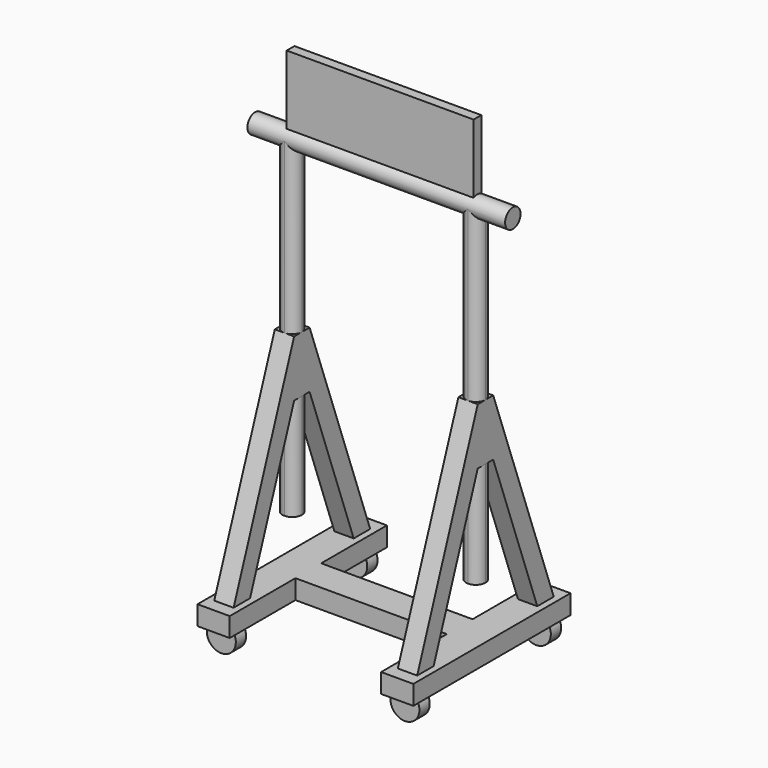
from build123d import *

# Parameters (mm, degrees)
F2_DEPTH          = 3
F6_DEPTH          = 1.5
F9_DEPTH          = 26.2
F9_DEPTH_BACK     = 25
F10_R             = 1.5
F11_DEPTH         = 20
F13_R             = 2.25
F14_DEPTH         = 2
F14_COPIES2_COUNT = 2
F14_COPIES2_PITCH = 38.242646
F15_W             = 29
F15_H             = 11
F16_DEPTH         = 0.75


# Not quite as in the source:
# - a pattern or mirror of a feature is missing from the dataset's text; its kind, count and spacing are read off the source's solid


with BuildPart() as f2:
    # F1 (on offset) → F2 (new body)
    with BuildSketch(Plane.XY.offset(3.5)):
        Polygon((-11.75, -15.25), (-11.75, -2.5), (-11.75, 2.5), (-11.75, 15.25), (-16.75, 15.25), (-16.75, 0), (-16.75, -15.25), align=None)
        Polygon((0, -2.5), (11.75, -2.5), (11.75, 2.5), (0, 2.5), (-11.75, 2.5), (-11.75, -2.5), align=None)
        Polygon((16.75, -15.25), (16.75, 0), (16.75, 15.25), (11.75, 15.25), (11.75, 2.5), (11.75, -2.5), (11.75, -15.25), align=None)
    extrude(amount=F2_DEPTH)

    # F5 (on plane+point) → F6 (join, symmetric)
    with BuildSketch(Plane.YZ.offset(14.25)):
        Polygon((10.057664814, 6.5), (13.25, 6.5), (1.5, 38.8), (0, 38.8), (-1.5, 38.8), (-13.25, 6.5), (-10.057664814, 6.5), (-1.5, 30.0244743399), (0, 30.0244743399), (1.5, 30.0244743399), align=None)
    f6 = extrude(amount=F6_DEPTH, both=True)

    # F6_copies: F6 across plane
    add(f6.mirror(Plane(origin=(0, 0, 0), x_dir=(0, 0, -1), z_dir=(-1, 0, 0))))

    # F8 (on face) → F9 (join, two sides)
    with BuildSketch(Plane.XY.offset(38.8)) as f9_sk:
        with BuildLine():
            ThreePointArc((14.25, -1.5), (15.3106601718, -1.0606601718), (15.75, 0))
            ThreePointArc((15.75, 0), (15.3106601718, 1.0606601718), (14.25, 1.5))
            ThreePointArc((14.25, 1.5), (13.1893398223, 1.0606601659), (12.75, -1.67e-08))
            ThreePointArc((12.75, -1.67e-08), (13.1893398341, -1.0606601777), (14.25, -1.5))
        make_face()
    f9 = extrude(amount=F9_DEPTH) + extrude(f9_sk.sketch, amount=-F9_DEPTH_BACK)

    # F9_copies: F9 across plane
    add(f9.mirror(Plane(origin=(0, 0, 0), x_dir=(0, 0, -1), z_dir=(-1, 0, 0))))

    # F10 (on Right) → F11 (join, symmetric)
    with BuildSketch(Plane.YZ):
        with Locations((0, 65)):
            Circle(F10_R)
    extrude(amount=F11_DEPTH, both=True)

    # F13 (on offset) → F14 (join)
    with BuildSketch(Plane.XZ.offset(13.75)):
        with Locations((14.25, 2.25)):
            Circle(F13_R)
    f14 = extrude(amount=-F14_DEPTH)

    # F14_copies: F14 across plane
    add(f14.mirror(Plane.ZX))

    # F14_copies1: F14 across plane
    add(f14.mirror(Plane(origin=(0, 0, 0), x_dir=(0, 0, -1), z_dir=(-1, 0, 0))))

    # F14_copies2: F14 ×2
    with Locations(*[Vector(-0.7452413135, 0.6667948595, 0) * (i * F14_COPIES2_PITCH) for i in range(1, F14_COPIES2_COUNT)]):
        add(f14)

    # F15 (on Front) → F16 (join, symmetric)
    with BuildSketch(Plane.XZ):
        with Locations((0, 71.5)):
            Rectangle(F15_W, F15_H)
    extrude(amount=F16_DEPTH, both=True)


solid = f2.part
